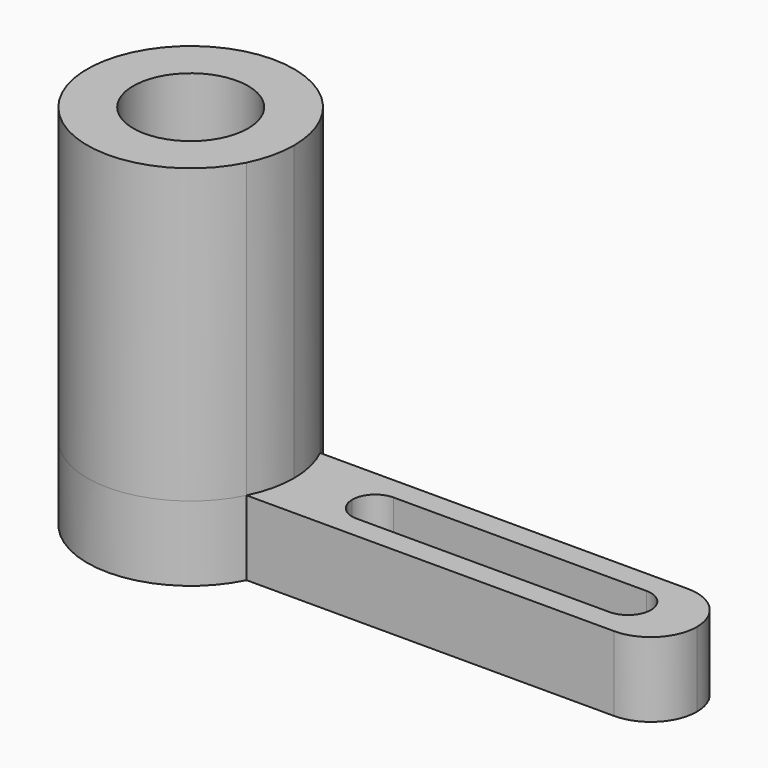
from build123d import *

# Parameters (mm, degrees)
F1_DEPTH    = 6.5
F3_DEPTH    = 25.5
F4_R        = 5
F5_DEPTH    = 32
F6_R        = 7.0774645673
F6_R_2      = 5
F7_DEPTH    = 12
F8_S5_R     = 5
F8_T6_DEPTH = 12


# Not quite as in the source:
# - a fillet or chamfer that OpenCascade refuses, or shapes differently, is made with other operations: its cross-section is extruded or revolved along the edge and cut away or added


with BuildPart() as f1:
    # F0 (on Top) → F1 (new body)
    with BuildSketch(Plane.XY):
        with BuildLine():
            Line((-28.7369439649, 4), (-60.7369439649, 4))
            ThreePointArc((-60.7369439649, 4), (-70.8534266602, 8.7624288794), (-77.7992017132, 0))
            ThreePointArc((-77.7992017132, 0), (-70.8534266602, -8.7624288794), (-60.7369439649, -4))
            Line((-60.7369439649, -4), (-28.7369439649, -4))
            ThreePointArc((-28.7369439649, -4), (-25.9085168402, -2.8284271247), (-24.7369439649, 0))
            ThreePointArc((-24.7369439649, 0), (-25.9085168402, 2.8284271247), (-28.7369439649, 4))
        make_face()
        with BuildLine():
            ThreePointArc((-54.7369439649, 0), (-54.1511575273, 1.4142135624), (-52.7369439649, 2))
            Line((-52.7369439649, 2), (-30.7369439649, 2))
            ThreePointArc((-30.7369439649, 2), (-29.3227304026, 1.4142135624), (-28.7369439649, 0))
            ThreePointArc((-28.7369439649, 0), (-29.3227304026, -1.4142135624), (-30.7369439649, -2))
            Line((-30.7369439649, -2), (-52.7369439649, -2))
            ThreePointArc((-52.7369439649, -2), (-54.1511575273, -1.4142135624), (-54.7369439649, 0))
        make_face(mode=Mode.SUBTRACT)
    extrude(amount=F1_DEPTH)

    # F2 (on face) → F3 (join)
    with BuildSketch(Plane.XY.offset(6.5)):
        with BuildLine():
            ThreePointArc((-60.7369439649, -4), (-60.0367728338, -2.0542249469), (-59.7992017132, 0))
            ThreePointArc((-59.7992017132, 0), (-60.0367728338, 2.0542249469), (-60.7369439649, 4))
            ThreePointArc((-60.7369439649, 4), (-77.7992017132, 0), (-60.7369439649, -4))
        make_face()
    extrude(amount=F3_DEPTH)

    # F4 (on face) → F5 (cut, through all)
    with BuildSketch(Plane.XY.offset(32)):
        with Locations((-68.7992017132, 0)):
            Circle(F4_R)
    extrude(amount=-F5_DEPTH, mode=Mode.SUBTRACT)

    # F6 (on face) → F7 (cut)
    with BuildSketch(Plane(origin=(0, 0, 0), x_dir=(1, 0, 0), z_dir=(0, 0, -1))):
        with Locations((-68.7992017132, 0)):
            Circle(F6_R)
        with Locations((-68.7992017132, 0)):
            Circle(F6_R_2, mode=Mode.SUBTRACT)
    extrude(amount=-F7_DEPTH, mode=Mode.SUBTRACT)

    # F8: chamfer of 5 on 1 edges, made by hand


with BuildPart() as f8_tool2:
    # F8_s3 → F8_t4 (revolve)
    with BuildSketch(Plane.XZ):
        Polygon((-61.721737146, 7), (-66.721737146, 12), (-61.721737146, 12), align=None)
    revolve(axis=Axis((-68.7992017132, 0, 12), (0, 0, -1)))

    # F8_s5 → F8_t6 (cut, symmetric)
    with BuildSketch(Plane.XY.offset(9.5)):
        with Locations((-68.7992017132, 0)):
            Circle(F8_S5_R)
    extrude(amount=F8_T6_DEPTH, both=True, mode=Mode.SUBTRACT)


with BuildPart() as f1_1:
    add(f1.part)

    # F8_t1: union F8_tool2
    add(f8_tool2.part)


solid = f1_1.part
